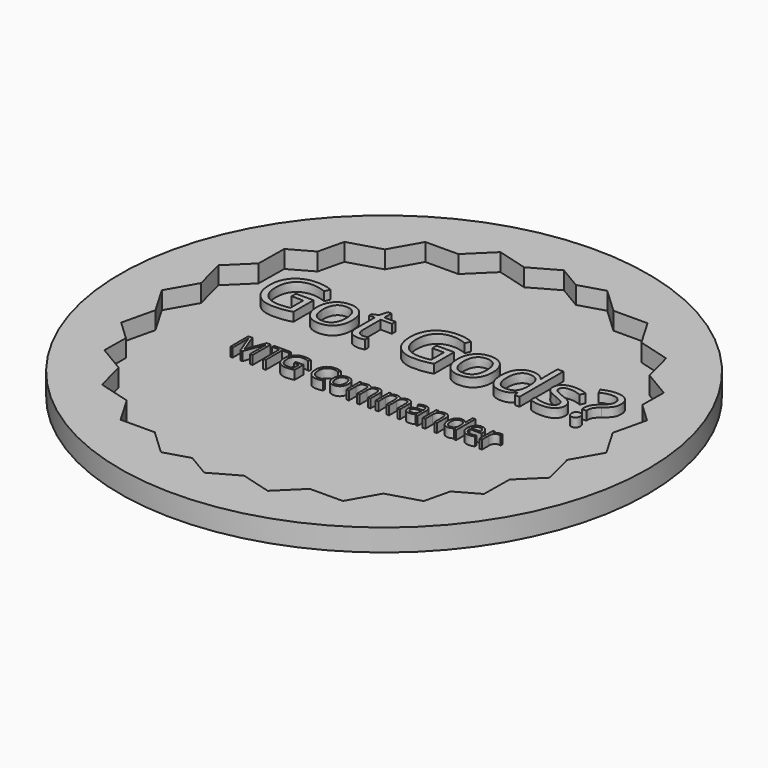
from build123d import *

# Parameters (mm, degrees)
F0_R           = 38.1
F1_DEPTH       = 3.175
F3_DEPTH       = 2.54
F4_TEXT_SIZE   = 4.5673184985
F4_TEXT_SIZE_2 = 10.435439698
F5_DEPTH       = 1.27


# Not quite as in the source:
# - Text() gives the source's letters only with a copy of the font that has no kerning and outlines rounded to 1/6400 em; it was checked with that copy


with BuildPart() as f1:
    # F0 (on Top) → F1 (new body)
    with BuildSketch(Plane.XY):
        Circle(F0_R)
    extrude(amount=F1_DEPTH)

    # F2 (on face) → F3 (cut)
    with BuildSketch(Plane.XY.offset(3.175)):
        Polygon((-16.7539807155, -22.2307116947), (-20.2813434379, -20.1346489786), (-18.2313309667, -23.6422477825), (-14.0041852642, -24.8207506786), align=None)
        Polygon((-15.8280923204, -27.7542213045), (-10.9174468457, -27.7281570579), (-14.0041852642, -24.8207506786), (-18.2313309667, -23.6422477825), align=None)
        Polygon((-7.5328270782, -27.7101925021), (-3.7128362491, -27.6899171262), (-10.9733600143, -25.6657265999), align=None)
        Polygon((0.2854385279, -28.8046121795), (-3.7128362491, -27.6899171262), (-7.5328270782, -27.7101925021), (-3.6848346955, -29.9967827964), align=None)
        Polygon((3.5707460553, -29.7205362351), (7.2964457928, -27.6314831294), (4.1364409877, -27.6482554956), (0.2854385279, -28.8046121795), align=None)
        Polygon((11.3591216989, -27.6099196532), (7.2964457928, -27.6314831294), (3.5707460553, -29.7205362351), (7.9575307916, -30.9435455373), align=None)
        Polygon((14.4933079966, -24.5383555374), (10.875370714, -25.6247287615), (7.2964457928, -27.6314831294), (11.3591216989, -27.6099196532), align=None)
        Polygon((16.1218145518, -27.5846406951), (18.5545649894, -23.3188648418), (14.4933079966, -24.5383555374), (11.3591216989, -27.6099196532), align=None)
        Polygon((21.8758711357, 17.4063907244), (20.2813434379, 20.1346489786), (16.7539807155, 22.2307116947), align=None)
        Polygon((20.2313171115, -20.3787158631), (22.1237535355, -17.0603690749), (16.7404912349, -22.3360718372), align=None)
        Polygon((25.0882451575, -14.1551090734), (22.1237535355, -17.0603690749), (20.2313171115, -20.3787158631), (24.1355585858, -18.1895518532), align=None)
        Polygon((27.5241124213, -11.7679113232), (27.5777892307, -7.4968341508), (26.0123121234, -10.2418647712), (25.0882451575, -14.1551090734), align=None)
        Polygon((29.5904526656, -3.9676718707), (27.5777892307, -7.4968341508), (27.5241124213, -11.7679113232), (30.7766619143, -8.5803489518), align=None)
        Polygon((28.4974932607, 0.2823951412), (27.6293514295, -3.3940170668), (27.5777892307, -7.4968341508), (29.5904526656, -3.9676718707), align=None)
        Polygon((31.9499068721, 0.1695806094), (29.4720118351, 4.4092922161), (28.4974932607, 0.2823951412), (29.5904526656, -3.9676718707), align=None)
        Polygon((27.7641441897, 7.331476639), (25.8365897845, 10.6295480513), (27.7138512493, 3.3296547627), align=None)
        Polygon((24.8028066296, 14.6495031061), (25.8365897845, 10.6295480513), (27.7641441897, 7.331476639), (27.8203932812, 11.8072309432), align=None)
        Polygon((23.953366366, 17.9526249119), (20.2813434379, 20.1346489786), (21.8758711357, 17.4063907244), (24.8028066296, 14.6495031061), align=None)
        Polygon((22.8191311227, 22.3631965856), (18.2313309667, 23.6422477825), (20.2813434379, 20.1346489786), (23.953366366, 17.9526249119), align=None)
        Polygon((20.2813434379, 20.1346489786), (18.2313309667, 23.6422477825), (14.0041852642, 24.8207506786), (16.7539807155, 22.2307116947), align=None)
        Polygon((18.2313309667, 23.6422477825), (15.8280923204, 27.7542213045), (10.9174468457, 27.7281570579), (14.0041852642, 24.8207506786), align=None)
        Polygon((3.7128362491, 27.6899171262), (7.5328270782, 27.7101925021), (3.6848346955, 29.9967827964), (-0.2854385279, 28.8046121795), align=None)
        Polygon((-7.2964457928, 27.6314831294), (-4.1364409877, 27.6482554956), (-0.2854385279, 28.8046121795), (-3.5707460553, 29.7205362351), align=None)
        Polygon((10.9733600143, 25.6657265999), (7.5328270782, 27.7101925021), (3.7128362491, 27.6899171262), align=None)
        Polygon((-10.875370714, 25.6247287615), (-7.2964457928, 27.6314831294), (-11.3591216989, 27.6099196532), (-14.4933079966, 24.5383555374), align=None)
        Polygon((-11.3591216989, 27.6099196532), (-7.2964457928, 27.6314831294), (-3.5707460553, 29.7205362351), (-7.9575307916, 30.9435455373), align=None)
        Polygon((-14.4933079966, 24.5383555374), (-11.3591216989, 27.6099196532), (-16.1218145518, 27.5846406951), (-18.5545649894, 23.3188648418), align=None)
        Polygon((-22.1237535355, 17.0603690749), (-16.7404912349, 22.3360718372), (-20.2313171115, 20.3787158631), align=None)
        Polygon((-22.1237535355, 17.0603690749), (-20.2313171115, 20.3787158631), (-24.1355585858, 18.1895518532), (-25.0882451575, 14.1551090734), align=None)
        Polygon((-27.5777892307, 7.4968341508), (-26.0123121234, 10.2418647712), (-25.0882451575, 14.1551090734), (-27.5241124213, 11.7679113232), align=None)
        Polygon((-29.5904526656, 3.9676718707), (-27.5777892307, 7.4968341508), (-27.5241124213, 11.7679113232), (-30.7766619143, 8.5803489518), align=None)
        Polygon((-27.6293514295, 3.3940170668), (-27.5777892307, 7.4968341508), (-29.5904526656, 3.9676718707), (-28.4974932607, -0.2823951412), align=None)
        Polygon((-28.4974932607, -0.2823951412), (-29.5904526656, 3.9676718707), (-31.9499068721, -0.1695806094), (-29.4720118351, -4.4092922161), align=None)
        Polygon((-25.8365897845, -10.6295480513), (-27.7138512493, -3.3296547627), (-27.7641441897, -7.331476639), align=None)
        Polygon((-20.2813434379, -20.1346489786), (-21.8758711357, -17.4063907244), (-24.8028066296, -14.6495031061), (-23.953366366, -17.9526249119), align=None)
        Polygon((-25.8365897845, -10.6295480513), (-27.7641441897, -7.331476639), (-27.8203932812, -11.8072309432), (-24.8028066296, -14.6495031061), align=None)
        Polygon((-24.8028066296, -14.6495031061), (-27.8203932812, -11.8072309432), (-27.8683882635, -15.6262037078), (-23.953366366, -17.9526249119), align=None)
        Polygon((-27.8203932812, -11.8072309432), (-27.7641441897, -7.331476639), (-29.4720118351, -4.4092922161), (-30.6005813396, -9.1885650892), align=None)
        Polygon((-27.7641441897, -7.331476639), (-27.7138512493, -3.3296547627), (-28.4974932607, -0.2823951412), (-29.4720118351, -4.4092922161), align=None)
        Polygon((-27.7138512493, -3.3296547627), (-27.6293514295, 3.3940170668), (-28.4974932607, -0.2823951412), align=None)
        Polygon((-27.6293514295, 3.3940170668), (-26.0123121234, 10.2418647712), (-27.5777892307, 7.4968341508), align=None)
        Polygon((-26.0123121234, 10.2418647712), (-22.1237535355, 17.0603690749), (-25.0882451575, 14.1551090734), align=None)
        Polygon((-25.0882451575, 14.1551090734), (-24.1355585858, 18.1895518532), (-27.4668835074, 16.3216303448), (-27.5241124213, 11.7679113232), align=None)
        Polygon((-24.1355585858, 18.1895518532), (-20.2313171115, 20.3787158631), (-18.5545649894, 23.3188648418), (-23.2578214614, 21.9065982661), align=None)
        Polygon((7.5328270782, 27.7101925021), (10.9174468457, 27.7281570579), (7.3427598783, 31.0951633553), (3.6848346955, 29.9967827964), align=None)
        Polygon((-0.2854385279, 28.8046121795), (3.6848346955, 29.9967827964), (0.4015047561, 31.9478340526), (-3.5707460553, 29.7205362351), align=None)
        Polygon((-4.1364409877, 27.6482554956), (3.7128362491, 27.6899171262), (-0.2854385279, 28.8046121795), align=None)
        Polygon((-10.875370714, 25.6247287615), (-4.1364409877, 27.6482554956), (-7.2964457928, 27.6314831294), align=None)
        Polygon((-20.2313171115, 20.3787158631), (-16.7404912349, 22.3360718372), (-14.4933079966, 24.5383555374), (-18.5545649894, 23.3188648418), align=None)
        Polygon((27.8203932812, 11.8072309432), (27.7641441897, 7.331476639), (29.4720118351, 4.4092922161), (30.6005813396, 9.1885650892), align=None)
        Polygon((27.8683882635, 15.6262037078), (23.953366366, 17.9526249119), (24.8028066296, 14.6495031061), (27.8203932812, 11.8072309432), align=None)
        Polygon((29.4720118351, 4.4092922161), (27.7641441897, 7.331476639), (27.7138512493, 3.3296547627), (28.4974932607, 0.2823951412), align=None)
        Polygon((27.4668835074, -16.3216303448), (27.5241124213, -11.7679113232), (25.0882451575, -14.1551090734), (24.1355585858, -18.1895518532), align=None)
        Polygon((24.1355585858, -18.1895518532), (20.2313171115, -20.3787158631), (18.5545649894, -23.3188648418), (23.2578214614, -21.9065982661), align=None)
        Polygon((18.5545649894, -23.3188648418), (20.2313171115, -20.3787158631), (16.7404912349, -22.3360718372), (14.4933079966, -24.5383555374), align=None)
        Polygon((-0.4015047561, -31.9478340526), (3.5707460553, -29.7205362351), (0.2854385279, -28.8046121795), (-3.6848346955, -29.9967827964), align=None)
        Polygon((-3.6848346955, -29.9967827964), (-7.5328270782, -27.7101925021), (-10.9174468457, -27.7281570579), (-7.3427598783, -31.0951633553), align=None)
        Polygon((-10.9174468457, -27.7281570579), (-7.5328270782, -27.7101925021), (-10.9733600143, -25.6657265999), (-14.0041852642, -24.8207506786), align=None)
        Polygon((14.0041852642, 24.8207506786), (10.9174468457, 27.7281570579), (7.5328270782, 27.7101925021), (10.9733600143, 25.6657265999), align=None)
        Polygon((25.8365897845, 10.6295480513), (21.8758711357, 17.4063907244), (16.7539807155, 22.2307116947), (10.9733600143, 25.6657265999), (3.7128362491, 27.6899171262), (-4.1364409877, 27.6482554956), (-10.875370714, 25.6247287615), (-16.7404912349, 22.3360718372), (-22.1237535355, 17.0603690749), (-26.0123121234, 10.2418647712), (-27.6293514295, 3.3940170668), (-27.7138512493, -3.3296547627), (-25.8365897845, -10.6295480513), (-21.8758711357, -17.4063907244), (-16.7539807155, -22.2307116947), (-10.9733600143, -25.6657265999), (-3.7128362491, -27.6899171262), (4.1364409877, -27.6482554956), (10.875370714, -25.6247287615), (16.7404912349, -22.3360718372), (22.1237535355, -17.0603690749), (26.0123121234, -10.2418647712), (27.6293514295, -3.3940170668), (27.7138512493, 3.3296547627), align=None)
        Polygon((27.5777892307, -7.4968341508), (27.6293514295, -3.3940170668), (26.0123121234, -10.2418647712), align=None)
        Polygon((25.0882451575, -14.1551090734), (26.0123121234, -10.2418647712), (22.1237535355, -17.0603690749), align=None)
        Polygon((7.2964457928, -27.6314831294), (10.875370714, -25.6247287615), (4.1364409877, -27.6482554956), align=None)
        Polygon((14.4933079966, -24.5383555374), (16.7404912349, -22.3360718372), (10.875370714, -25.6247287615), align=None)
        Polygon((0.2854385279, -28.8046121795), (4.1364409877, -27.6482554956), (-3.7128362491, -27.6899171262), align=None)
        Polygon((-14.0041852642, -24.8207506786), (-10.9733600143, -25.6657265999), (-16.7539807155, -22.2307116947), align=None)
        Polygon((-18.2313309667, -23.6422477825), (-20.2813434379, -20.1346489786), (-23.953366366, -17.9526249119), (-22.8191311227, -22.3631965856), align=None)
        Polygon((-21.8758711357, -17.4063907244), (-25.8365897845, -10.6295480513), (-24.8028066296, -14.6495031061), align=None)
        Polygon((-16.7539807155, -22.2307116947), (-21.8758711357, -17.4063907244), (-20.2813434379, -20.1346489786), align=None)
        Polygon((16.7539807155, 22.2307116947), (14.0041852642, 24.8207506786), (10.9733600143, 25.6657265999), align=None)
        Polygon((-16.7404912349, 22.3360718372), (-10.875370714, 25.6247287615), (-14.4933079966, 24.5383555374), align=None)
        Polygon((24.8028066296, 14.6495031061), (21.8758711357, 17.4063907244), (25.8365897845, 10.6295480513), align=None)
        Polygon((28.4974932607, 0.2823951412), (27.7138512493, 3.3296547627), (27.6293514295, -3.3940170668), align=None)
    extrude(amount=-F3_DEPTH, mode=Mode.SUBTRACT)

    # F4 (on face) → F5 (join)
    with BuildSketch(Plane.XY.offset(0.635)):
        with Locations((-19.2841845094, -4.2086550584)):
            Text('MTG Commander', F4_TEXT_SIZE, font='Open Sans', text_align=(TextAlign.LEFT, TextAlign.BOTTOM))
        with Locations((-25.4309938464, 6.6114990041)):
            Text('Got Gods?', F4_TEXT_SIZE_2, font='Open Sans', text_align=(TextAlign.LEFT, TextAlign.BOTTOM))
    extrude(amount=F5_DEPTH)


solid = f1.part
